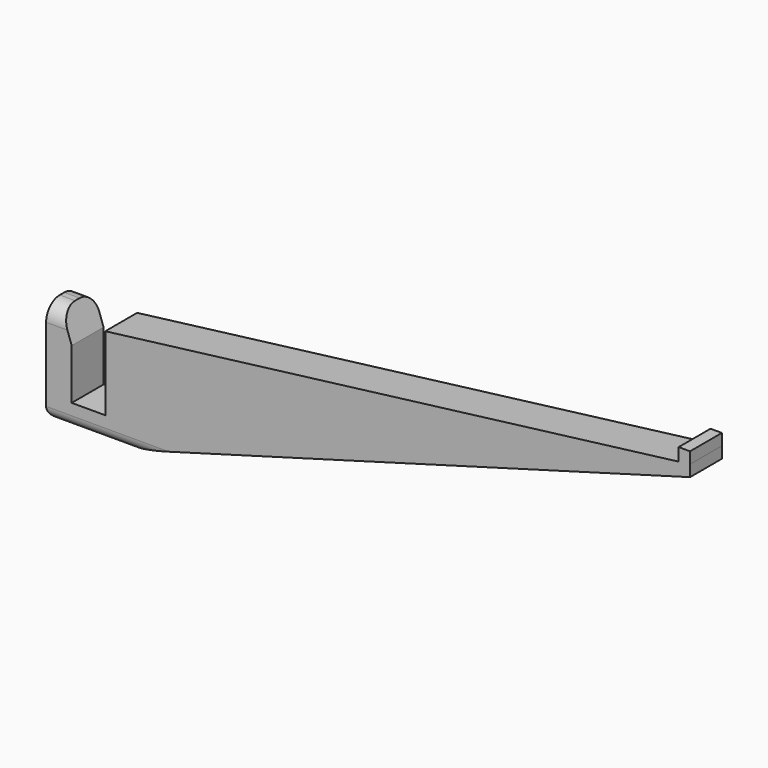
from build123d import *

# Parameters (mm, degrees)
F1_DEPTH = 3.5
F2_R     = 3
F3_R     = 2


with BuildPart() as f1:
    # F0 (on Front) → F1 (new body, symmetric)
    with BuildSketch(Plane.XZ):
        Polygon((-28.2374123681, -10.7569159286), (-34.1374123681, -10.7569159286), (-34.1374123681, -1.9036901649), (-35.9374123681, 3.2430840714), (-37.7374123681, 3.2430840714), (-38.6374123681, 3.2430840714), (-38.6374123681, -1.7569159286), (-38.6374123681, -14.7569159286), (-24.1374123681, -14.7569159286), (74.5055291286, 13.0817538947), (74.5024305759, 15.0817514944), (74.5024305759, 17.0817514944), (72.5024305759, 17.0817514944), (72.5024305759, 14.8318257197), (-28.2374123681, 2.2430840714), (-28.2374123681, -1.7569159286), align=None)
    extrude(amount=F1_DEPTH, both=True)

    # F2
    f2_edges = [f1.edges().sort_by_distance(p)[0] for p in [
        (-37.287412, 3.5, 3.243084),
        (-37.287412, -3.5, 3.243084),
    ]]
    fillet(f2_edges, radius=F2_R)

    # F3
    f3_edges = [f1.edges().sort_by_distance(p)[0] for p in [
        (-38.637412, 0, -14.756916),
        (-31.387412, 3.5, -14.756916),
        (-24.137412, 0, -14.756916),
        (-31.387412, -3.5, -14.756916),
    ]]
    fillet(f3_edges, radius=F3_R)


solid = f1.part
